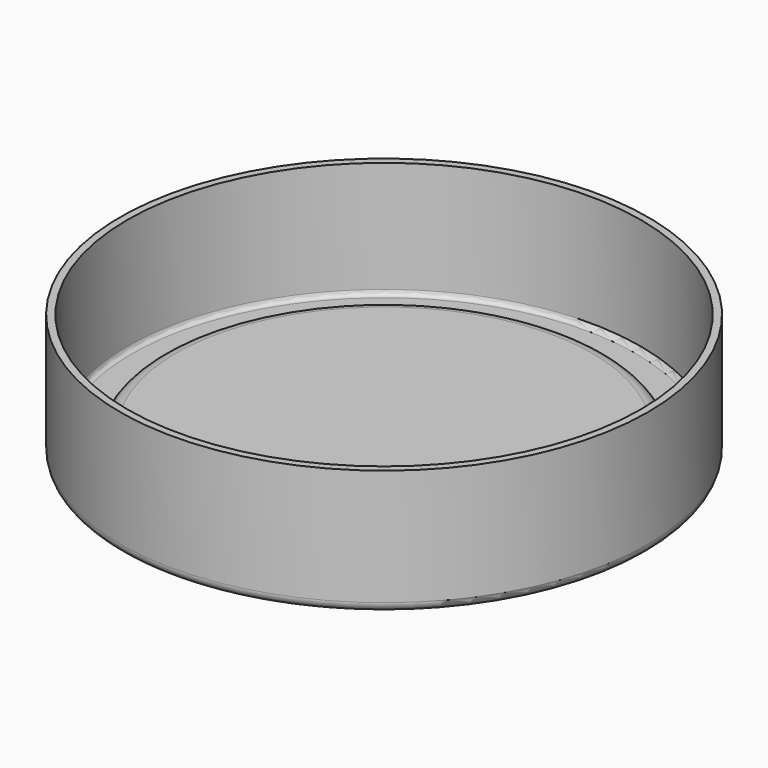
from build123d import *

# Parameters (mm, degrees)
F0_R     = 27.25
F1_DEPTH = 13
F2_R     = 26.5
F3_DEPTH = 12
F4_R     = 23
F5_DEPTH = 1.5
F6_R     = 1.49999
F7_R     = 1
F8_R     = 0.5


# Not quite as in the source:
# - a fillet or chamfer is up to 0.001 mm smaller than in the source, because OpenCascade refuses the exact size


with BuildPart() as f1:
    # F0 (on Top) → F1 (new body)
    with BuildSketch(Plane.XY):
        Circle(F0_R)
    extrude(amount=F1_DEPTH)

    # F2 (on face) → F3 (cut)
    with BuildSketch(Plane.XY.offset(13)):
        Circle(F2_R)
    extrude(amount=-F3_DEPTH, mode=Mode.SUBTRACT)

    # F4 (on face) → F5 (join)
    with BuildSketch(Plane.XY.offset(1)):
        Circle(F4_R)
    extrude(amount=F5_DEPTH)

    # F6 (radius 1.5 in the source; OpenCascade refuses exactly that, so slightly less here)
    f6_edges = [f1.edges().sort_by_distance(p)[0] for p in [
        (-23, 0, 2.5),
    ]]
    fillet(f6_edges, radius=F6_R)

    # F7
    f7_edges = [f1.edges().sort_by_distance(p)[0] for p in [
        (-27.25, 0, 0),
    ]]
    fillet(f7_edges, radius=F7_R)

    # F8
    f8_edges = [f1.edges().sort_by_distance(p)[0] for p in [
        (-26.5, 0, 1),
    ]]
    fillet(f8_edges, radius=F8_R)


solid = f1.part
